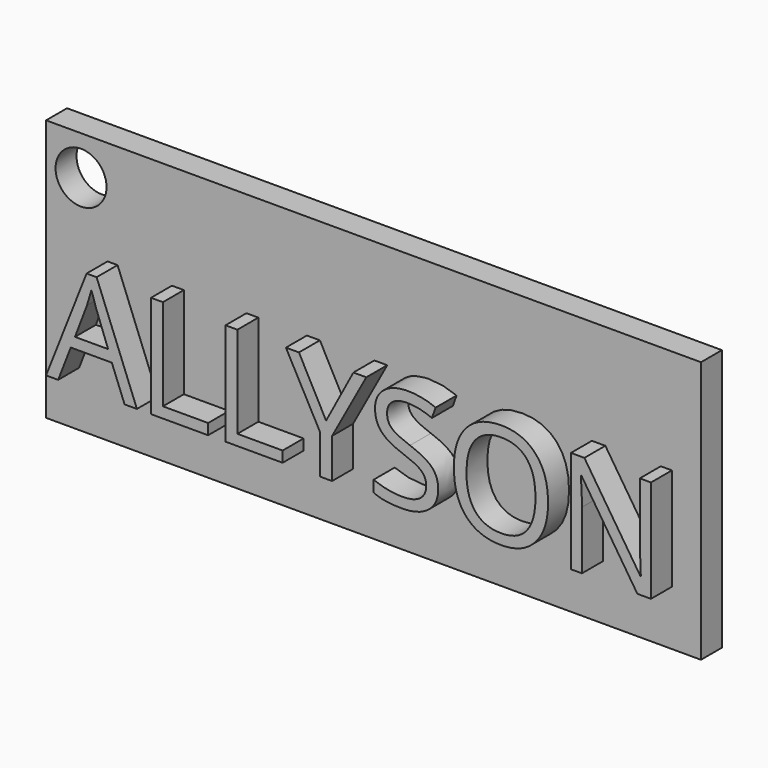
from build123d import *

# Parameters (mm, degrees)
F1_TEXT_SIZE = 10.9583333333
F2_DEPTH     = 4
F3_W         = 50
F3_H         = 20
F4_DEPTH     = 2
F5_R         = 1.9453301094
F6_DEPTH     = 2.0010001


# Not quite as in the source:
# - Text() gives the source's letters only with a copy of the font that has no kerning and outlines rounded to 1/6400 em; it was checked with that copy


with BuildPart() as f2:
    # F1 (on Front) → F2 (new body)
    with BuildSketch(Plane.XZ):
        with Locations((-8.0295437539, 19.7480395436)):
            Text('ALLYSON', F1_TEXT_SIZE, font='Open Sans', text_align=(TextAlign.LEFT, TextAlign.BOTTOM))
    extrude(amount=F2_DEPTH)


with BuildPart() as f4:
    # F3 (on Front) → F4 (new body)
    with BuildSketch(Plane.XZ):
        with Locations((15.3697548434, 25.5600989237)):
            Rectangle(F3_W, F3_H)
    extrude(amount=F4_DEPTH)

    # F5 (on face) → F6 (cut, through all)
    with BuildSketch(Plane.XZ.offset(2)):
        with Locations((-6.9613405503, 32.5743630528)):
            Circle(F5_R)
    extrude(amount=-F6_DEPTH, mode=Mode.SUBTRACT)


solid = Compound([f2.part, f4.part])
